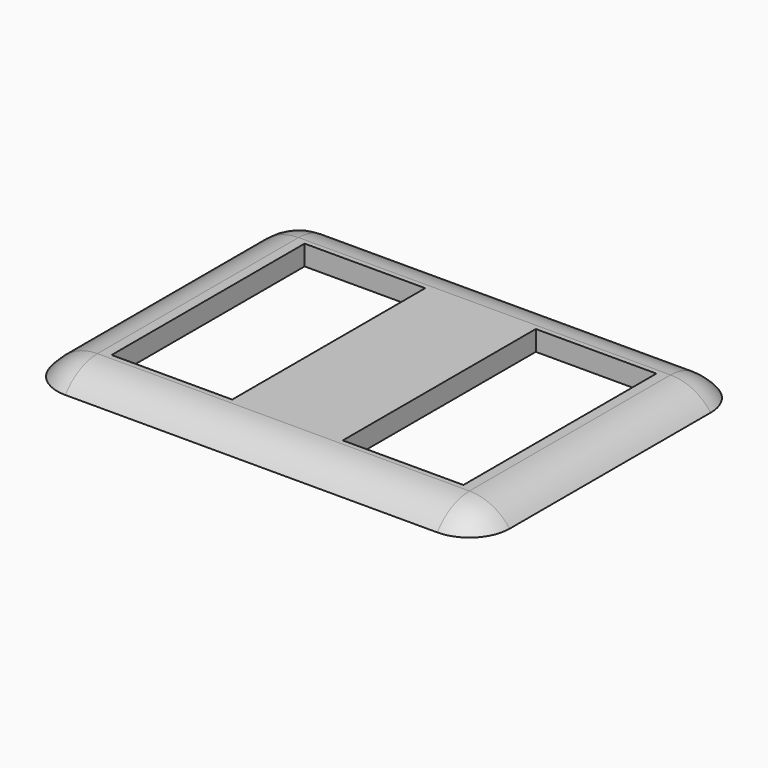
from build123d import *

# Parameters (mm, degrees)
F1_W        = 45
F1_H        = 35
F1_W_2      = 12
F1_H_2      = 24
F2_DEPTH    = 2
F3_T1_DEPTH = 55
F4_T1_DEPTH = 55
F5_T1_DEPTH = 37
F5_T4_ANGLE = 196.3896000127
F5_T6_ANGLE = 196.3896000127
F6_T1_DEPTH = 37
F6_T4_ANGLE = 196.3896000127
F6_T6_ANGLE = 196.3896000127


# Not quite as in the source:
# - a fillet or chamfer that OpenCascade refuses, or shapes differently, is made with other operations: its cross-section is extruded or revolved along the edge and cut away or added


with BuildPart() as f2:
    # F1 (on face) → F2 (new body)
    with BuildSketch(Plane.XY):
        with Locations((-7.2387225181, -9.9369412684)):
            Rectangle(F1_W, F1_H)
        with Locations((-18.7387225181, -9.9369412684)):
            Rectangle(F1_W_2, F1_H_2, mode=Mode.SUBTRACT)
        with Locations((4.2612774819, -9.9369412684)):
            Rectangle(F1_W_2, F1_H_2, mode=Mode.SUBTRACT)
    extrude(amount=F2_DEPTH)

    # F3: fillet of radius 5 on 1 edges, made by hand

    # F3_s2 → F3_t1 (cut)
    with BuildSketch(Plane.XZ.offset(-17.5630587316)):
        with BuildLine():
            ThreePointArc((-29.7387225181, 0), (-27.9747904956, 1.472135955), (-25.7387225181, 2))
            Line((-25.7387225181, 2), (-29.7387225181, 2))
            Line((-29.7387225181, 2), (-29.7387225181, 0))
        make_face()
    extrude(amount=F3_T1_DEPTH, mode=Mode.SUBTRACT)

    # F4: fillet of radius 5 on 1 edges, made by hand

    # F4_s2 → F4_t1 (cut)
    with BuildSketch(Plane.XZ.offset(-17.5630587316)):
        with BuildLine():
            ThreePointArc((15.2612774819, 0), (13.4973454594, 1.472135955), (11.2612774819, 2))
            Line((11.2612774819, 2), (15.2612774819, 2))
            Line((15.2612774819, 2), (15.2612774819, 0))
        make_face()
    extrude(amount=F4_T1_DEPTH, mode=Mode.SUBTRACT)

    # F5: fillet of radius 5 on 1 edges, made by hand

    # F5_s2 → F5_t1 (cut)
    with BuildSketch(Plane.YZ.offset(-25.7387225181)):
        with BuildLine():
            ThreePointArc((-27.4369412684, -3), (-25.9724751743, 0.5355339059), (-22.4369412684, 2))
            Line((-22.4369412684, 2), (-27.4369412684, 2))
            Line((-27.4369412684, 2), (-27.4369412684, -3))
        make_face()
    extrude(amount=F5_T1_DEPTH, mode=Mode.SUBTRACT)

    # F5_s3 → F5_t4 (revolve, cut)
    with BuildSketch(Plane(origin=(-24.5015511946, 0, -7.2063663149), x_dir=(0, 1, 0), z_dir=(0.9593652077, 0, 0.2821673233))):
        with BuildLine():
            ThreePointArc((-22.4369412684, -0.615469186), (-25.9724751743, 0.848996908), (-27.4369412684, 4.384530814))
            Line((-27.4369412684, 4.384530814), (-27.4369412684, -0.615469186))
            Line((-27.4369412684, -0.615469186), (-22.4369412684, -0.615469186))
        make_face()
    revolve(axis=Axis((-25.7387225181, -27.4369412684, -3), (0, 1, 0)), revolution_arc=F5_T4_ANGLE, mode=Mode.SUBTRACT)

    # F5_s5 → F5_t6 (revolve, cut)
    with BuildSketch(Plane.YZ.offset(11.2612774819)):
        with BuildLine():
            ThreePointArc((-22.4369412684, 2), (-25.9724751743, 0.5355339059), (-27.4369412684, -3))
            Line((-27.4369412684, -3), (-27.4369412684, 2))
            Line((-27.4369412684, 2), (-22.4369412684, 2))
        make_face()
    revolve(axis=Axis((11.2612774819, -27.4369412684, -3), (0, 1, 0)), revolution_arc=F5_T6_ANGLE, mode=Mode.SUBTRACT)

    # F6: fillet of radius 5 on 1 edges, made by hand

    # F6_s2 → F6_t1 (cut)
    with BuildSketch(Plane.YZ.offset(-25.7387225181)):
        with BuildLine():
            ThreePointArc((7.5630587316, -3), (6.0985926376, 0.5355339059), (2.5630587316, 2))
            Line((2.5630587316, 2), (7.5630587316, 2))
            Line((7.5630587316, 2), (7.5630587316, -3))
        make_face()
    extrude(amount=F6_T1_DEPTH, mode=Mode.SUBTRACT)

    # F6_s3 → F6_t4 (revolve, cut)
    with BuildSketch(Plane.YZ.offset(11.2612774819)):
        with BuildLine():
            ThreePointArc((7.5630587316, -3), (6.0985926376, 0.5355339059), (2.5630587316, 2))
            Line((2.5630587316, 2), (7.5630587316, 2))
            Line((7.5630587316, 2), (7.5630587316, -3))
        make_face()
    revolve(axis=Axis((11.2612774819, 7.5630587316, -3), (0, 1, 0)), revolution_arc=F6_T4_ANGLE, mode=Mode.SUBTRACT)

    # F6_s5 → F6_t6 (revolve, cut)
    with BuildSketch(Plane(origin=(-24.5015511946, 0, -7.2063663149), x_dir=(0, 1, 0), z_dir=(0.9593652077, 0, 0.2821673233))):
        with BuildLine():
            ThreePointArc((2.5630587316, -0.615469186), (6.0985926376, 0.848996908), (7.5630587316, 4.384530814))
            Line((7.5630587316, 4.384530814), (7.5630587316, -0.615469186))
            Line((7.5630587316, -0.615469186), (2.5630587316, -0.615469186))
        make_face()
    revolve(axis=Axis((-25.7387225181, 7.5630587316, -3), (0, 1, 0)), revolution_arc=F6_T6_ANGLE, mode=Mode.SUBTRACT)


solid = f2.part
